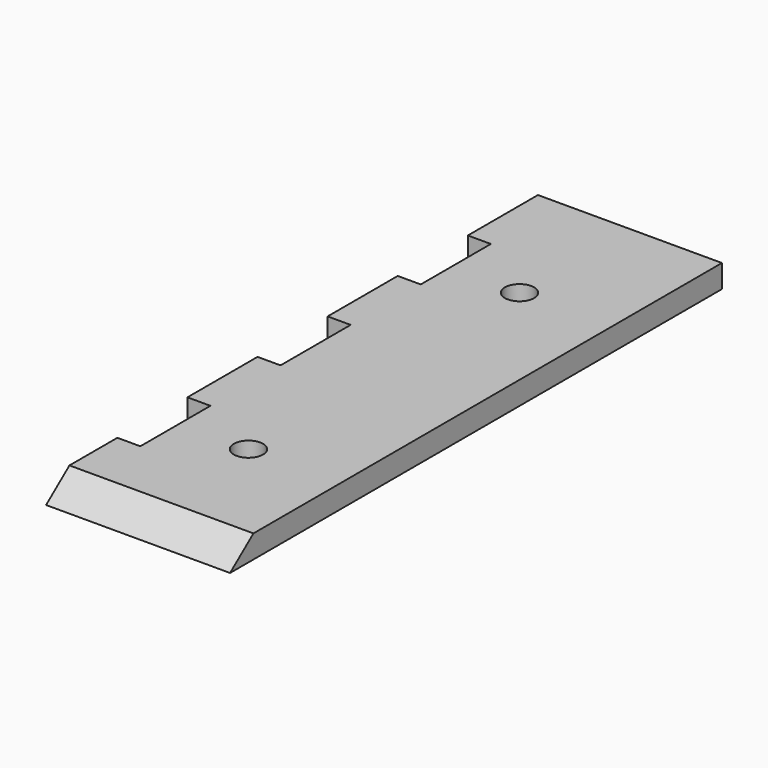
from build123d import *

# Parameters (mm, degrees)
F0_W     = 40
F0_H     = 133.6666618
F1_DEPTH = 5
F2_W     = 5
F2_H     = 19.05
F3_DEPTH = 25.4
F5_DEPTH = 40.001
F6_R     = 3.175
F7_DEPTH = 25.4


# Not quite as in the source:
# - a feature names something its author has since deleted; it is built from what else it names


with BuildPart() as f1:
    # F0 (on Top) → F1 (new body)
    with BuildSketch(Plane.XY):
        with Locations((-34.4807878137, 41.8868735433)):
            Rectangle(F0_W, F0_H)
    extrude(amount=F1_DEPTH)

    # F2 (on face) → F3 (cut)
    with BuildSketch(Plane.XY.offset(5)):
        with Locations((-51.9807878137, 80.1452044433)):
            Rectangle(F2_W, F2_H)
        with Locations((-51.9807878137, 42.0452044433)):
            Rectangle(F2_W, F2_H)
        with Locations((-51.9807878137, 3.9452044433)):
            Rectangle(F2_W, F2_H)
    extrude(amount=-F3_DEPTH, mode=Mode.SUBTRACT)

    # F4 (on face) → F5 (cut, through all)
    with BuildSketch(Plane.YZ.offset(-14.4807878137)):
        Polygon((-24.9464573567, 5), (-24.9464573567, 0), (-18.5964573465, 5), align=None)
    extrude(amount=-F5_DEPTH, mode=Mode.SUBTRACT)

    # F6 (on face) → F7 (cut)
    with BuildSketch(Plane.XY.offset(5)):
        with Locations((-34.4807878137, 5.0535426433)):
            Circle(F6_R)
        with Locations((-34.4807878137, 78.7202044433)):
            Circle(F6_R)
    extrude(amount=-F7_DEPTH, mode=Mode.SUBTRACT)


with BuildPart() as f8_1:
    # F8: copy of F1
    add(f1.part)


solid = Compound([f1.part, f8_1.part])
